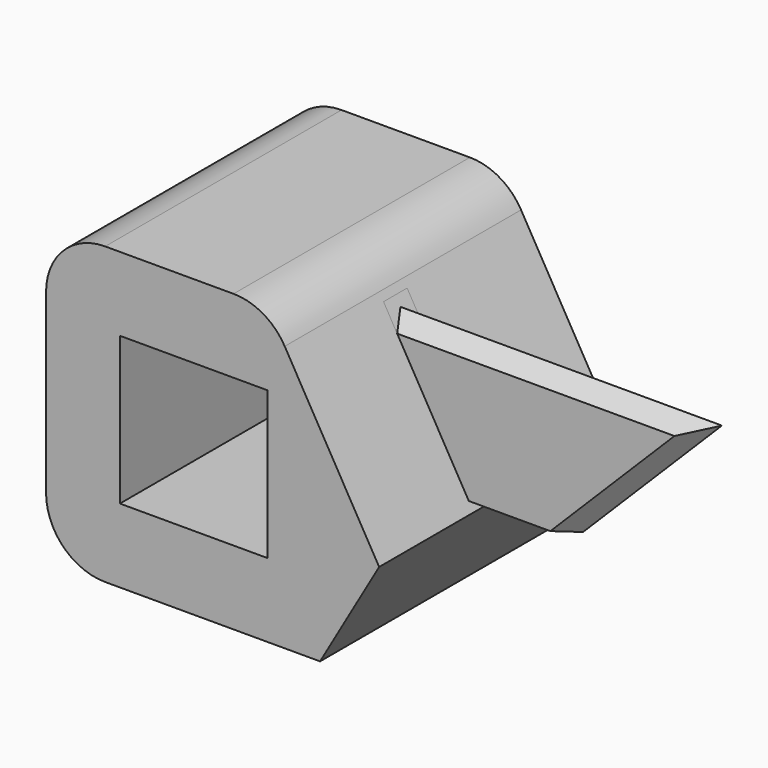
from build123d import *

# Parameters (mm, degrees)
F0_W        = 12.7
F0_H        = 12.7
F1_DEPTH    = 25.4
F4_DEPTH    = 2.54
F5_R        = 5.08
F6_SIZE     = 10.16
F7_T4_DEPTH = 40.3682325584
F7_T9_DEPTH = 40.3682325584
F8_T1_DEPTH = 25.5381499465


# Not quite as in the source:
# - a fillet or chamfer that OpenCascade refuses, or shapes differently, is made with other operations: its cross-section is extruded or revolved along the edge and cut away or added
# - a feature names something its author has since deleted; it is built from what else it names


with BuildPart() as f1:
    # F0 (on Front) → F1 (new body)
    with BuildSketch(Plane.XZ):
        Polygon((19.05, 25.4), (0, 25.4), (0, 0), (33.7146968374, 0), align=None)
        with Locations((12.7, 12.7)):
            Rectangle(F0_W, F0_H, mode=Mode.SUBTRACT)
    extrude(amount=F1_DEPTH)

    # F3 (on mid) → F4 (join)
    with BuildSketch(Plane.XZ.offset(12.7)):
        Polygon((50.8, 22.225), (20.8830871047, 22.225), (28.2154355234, 9.525), (38.1, 9.525), align=None)
    extrude(amount=F4_DEPTH)

    # F5
    f5_edges = [f1.edges().sort_by_distance(p)[0] for p in [
        (0, -12.7, 0),
        (0, -12.7, 25.4),
        (19.05, -12.7, 25.4),
    ]]
    fillet(f5_edges, radius=F5_R)

    # F6
    f6_edges = [f1.edges().sort_by_distance(p)[0] for p in [
        (33.714697, -12.7, 0),
    ]]
    chamfer(f6_edges, length=F6_SIZE)

    # F7: chamfer of 2.032 on 2 edges, made by hand


with BuildPart() as f7_tool2:
    # F7_s3 → F7_t4 (new body)
    with BuildSketch(Plane.YZ.offset(56.0256598315)):
        Polygon((-14.732, 22.225), (-12.7, 20.193), (-12.7, 22.225), align=None)
    extrude(amount=-F7_T4_DEPTH)

    split(bisect_by=Plane(origin=(25.2860226281, 0, 14.598891971), x_dir=(0, 1, 0), z_dir=(0.8660254038, 0, 0.5)), keep=Keep.TOP)


with BuildPart() as f1_1:
    add(f1.part)

    # F7_t1: cut F7_tool2
    add(f7_tool2.part, mode=Mode.SUBTRACT)


with BuildPart() as f7_tool7:
    # F7_s8 → F7_t9 (new body)
    with BuildSketch(Plane.YZ.offset(56.0256598315)):
        Polygon((-15.24, 20.193), (-13.208, 22.225), (-15.24, 22.225), align=None)
    extrude(amount=-F7_T9_DEPTH)

    split(bisect_by=Plane(origin=(25.2860226281, 0, 14.598891971), x_dir=(0, 1, 0), z_dir=(0.8660254038, 0, 0.5)), keep=Keep.TOP)


with BuildPart() as f1_2:
    add(f1_1.part)

    # F7_t6: cut F7_tool7
    add(f7_tool7.part, mode=Mode.SUBTRACT)

    # F8: chamfer of 2.032 on 2 edges, made by hand

    # F8_s2 → F8_t1 (cut)
    with BuildSketch(Plane(origin=(20.1174004969, 0, 20.1174004969), x_dir=(0, 1, 0), z_dir=(0.7071067812, 0, 0.7071067812))):
        Polygon((-12.7, -18.1735762724), (-14.732, -20.2055762724), (-12.7, -20.2055762724), align=None)
        Polygon((-15.24, -18.1735762724), (-13.208, -20.2055762724), (-15.24, -20.2055762724), align=None)
    extrude(amount=F8_T1_DEPTH, mode=Mode.SUBTRACT)


solid = f1_2.part
